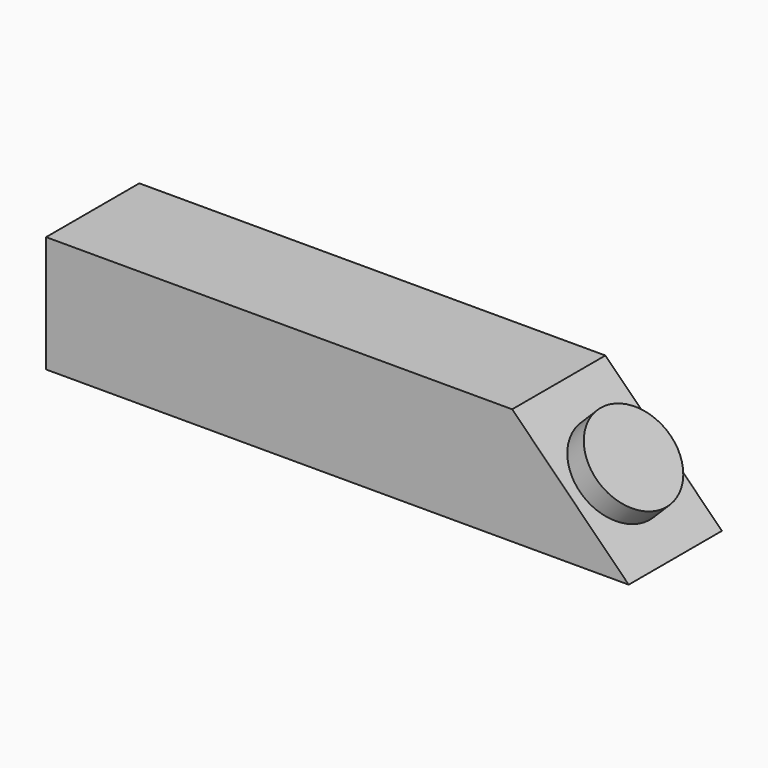
from build123d import *

# Parameters (mm, degrees)
F0_W     = 50
F0_H     = 10
F1_DEPTH = 10
F2_SIZE  = 9.99999
F3_R     = 4
F4_DEPTH = 2


# Not quite as in the source:
# - a fillet or chamfer is up to 0.001 mm smaller than in the source, because OpenCascade refuses the exact size


with BuildPart() as f1:
    # F0 (on Top) → F1 (new body)
    with BuildSketch(Plane.XY):
        with Locations((-21.3684089482, 18.842792958)):
            Rectangle(F0_W, F0_H)
    extrude(amount=F1_DEPTH)

    # F2 (size 10 in the source; OpenCascade refuses exactly that, so slightly less here)
    f2_edges = [f1.edges().sort_by_distance(p)[0] for p in [
        (3.631591, 18.842793, 10),
    ]]
    chamfer(f2_edges, length=F2_SIZE)

    # F3 (on face) → F4 (join)
    with BuildSketch(Plane(origin=(1.8157955259, 0, 1.8157955259), x_dir=(0, 1, 0), z_dir=(0.7071067812, 0, 0.7071067812))):
        with Locations((18.842792958, 4.5031451526)):
            Circle(F3_R)
    extrude(amount=F4_DEPTH)


solid = f1.part
